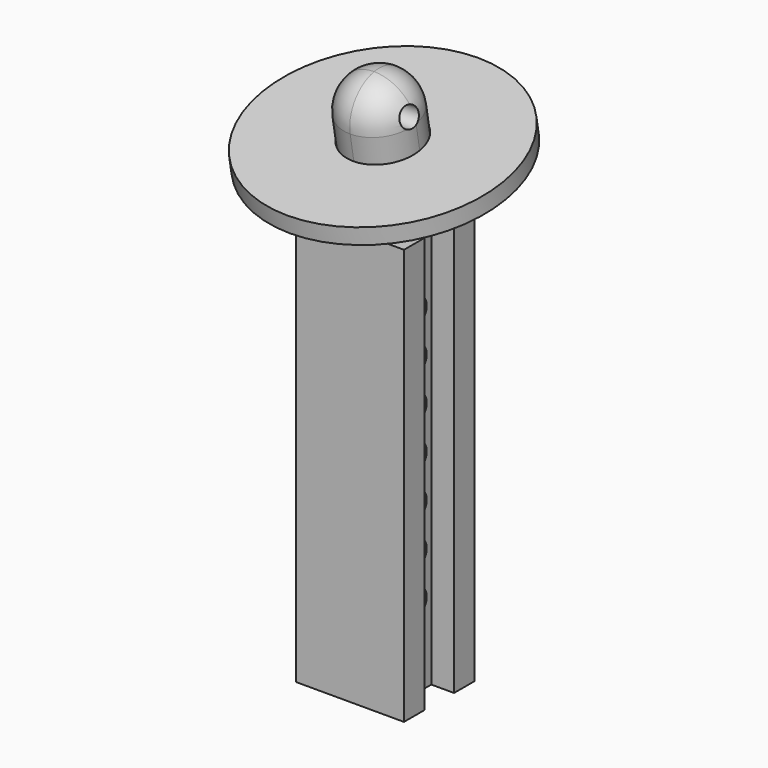
from build123d import *

# Parameters (mm, degrees)
F1_DEPTH     = 37.084
F3_DEPTH     = 25.4
F4_W         = 0.508
F4_H         = 3.302
F5_DEPTH     = 5.08
F6_T1_DEPTH  = 46.2057312575
F7_T1_DEPTH  = 13.1558517876
F7_T3_DEPTH  = 11.991388407
F9_DEPTH     = 7.112
F8_R         = 10.795
F10_DEPTH    = 1.524
F11_R        = 0.889
F12_DEPTH    = 25.4
F13_T1_DEPTH = 15.33525
F14_DEPTH    = 1.524
F15_T2_ANGLE = 89.9999999992
F15_T4_ANGLE = 90.0000000051
F15_T6_ANGLE = 89.9999999932
F15_T8_ANGLE = 89.9999999992


# Not quite as in the source:
# - a fillet or chamfer that OpenCascade refuses, or shapes differently, is made with other operations: its cross-section is extruded or revolved along the edge and cut away or added
# - a feature names something its author has since deleted; it is built from what else it names


with BuildPart() as f1:
    # F0 (on Top) → F1 (new body)
    with BuildSketch(Plane.XY):
        Polygon((13.1025131665, -0.5368698436), (3.4505131665, -0.5368698436), (3.4505131665, -2.8228698436), (5.4825131665, -2.8228698436), (5.4825131665, -6.1248698436), (3.4505131665, -6.1248698436), (3.4505131665, -8.4108698436), (13.1025131665, -8.4108698436), (13.1025131665, -6.1248698436), (11.0705131665, -6.1248698436), (11.0705131665, -2.8228698436), (13.1025131665, -2.8228698436), align=None)
    extrude(amount=F1_DEPTH)

    # F2 (on face) → F3 (cut)
    with BuildSketch(Plane.YZ.offset(11.0705131665)):
        with BuildLine():
            Line((-4.4738698436, 29.972), (-4.4738698436, 31.115))
            ThreePointArc((-4.4738698436, 31.115), (-5.6168698436, 29.972), (-4.4738698436, 28.829))
            Line((-4.4738698436, 28.829), (-4.4738698436, 29.972))
        make_face()
        with BuildLine():
            ThreePointArc((-4.4738698436, 28.829), (-3.6656467927, 29.1637769491), (-3.3308698436, 29.972))
            ThreePointArc((-3.3308698436, 29.972), (-3.6656467927, 30.7802230509), (-4.4738698436, 31.115))
            Line((-4.4738698436, 31.115), (-4.4738698436, 29.972))
            Line((-4.4738698436, 29.972), (-4.4738698436, 28.829))
        make_face()
        with BuildLine():
            ThreePointArc((-3.3308698436, 26.162), (-3.6656467927, 26.9702230509), (-4.4738698436, 27.305))
            Line((-4.4738698436, 27.305), (-4.4738698436, 26.162))
            Line((-4.4738698436, 26.162), (-4.4738698436, 25.019))
            ThreePointArc((-4.4738698436, 25.019), (-3.6656467927, 25.3537769491), (-3.3308698436, 26.162))
        make_face()
        with BuildLine():
            Line((-4.4738698436, 26.162), (-4.4738698436, 27.305))
            ThreePointArc((-4.4738698436, 27.305), (-5.6168698436, 26.162), (-4.4738698436, 25.019))
            Line((-4.4738698436, 25.019), (-4.4738698436, 26.162))
        make_face()
        with BuildLine():
            Line((-4.4738698436, 22.352), (-4.4738698436, 23.495))
            ThreePointArc((-4.4738698436, 23.495), (-5.6168698436, 22.352), (-4.4738698436, 21.209))
            Line((-4.4738698436, 21.209), (-4.4738698436, 22.352))
        make_face()
        with BuildLine():
            ThreePointArc((-3.3308698436, 22.352), (-3.6656467927, 23.1602230509), (-4.4738698436, 23.495))
            Line((-4.4738698436, 23.495), (-4.4738698436, 22.352))
            Line((-4.4738698436, 22.352), (-4.4738698436, 21.209))
            ThreePointArc((-4.4738698436, 21.209), (-3.6656467927, 21.5437769491), (-3.3308698436, 22.352))
        make_face()
        with BuildLine():
            ThreePointArc((-3.3308698436, 18.542), (-3.6656467927, 19.3502230509), (-4.4738698436, 19.685))
            Line((-4.4738698436, 19.685), (-4.4738698436, 18.542))
            Line((-4.4738698436, 18.542), (-4.4738698436, 17.399))
            ThreePointArc((-4.4738698436, 17.399), (-3.6656467927, 17.7337769491), (-3.3308698436, 18.542))
        make_face()
        with BuildLine():
            Line((-4.4738698436, 18.542), (-4.4738698436, 19.685))
            ThreePointArc((-4.4738698436, 19.685), (-5.6168698436, 18.542), (-4.4738698436, 17.399))
            Line((-4.4738698436, 17.399), (-4.4738698436, 18.542))
        make_face()
        with BuildLine():
            Line((-4.4738698436, 14.732), (-4.4738698436, 15.875))
            ThreePointArc((-4.4738698436, 15.875), (-5.6168698436, 14.732), (-4.4738698436, 13.589))
            Line((-4.4738698436, 13.589), (-4.4738698436, 14.732))
        make_face()
        with BuildLine():
            ThreePointArc((-3.3308698436, 14.732), (-3.6656467927, 15.5402230509), (-4.4738698436, 15.875))
            Line((-4.4738698436, 15.875), (-4.4738698436, 14.732))
            Line((-4.4738698436, 14.732), (-4.4738698436, 13.589))
            ThreePointArc((-4.4738698436, 13.589), (-3.6656467927, 13.9237769491), (-3.3308698436, 14.732))
        make_face()
        with BuildLine():
            Line((-4.4738698436, 10.922), (-4.4738698436, 9.779))
            ThreePointArc((-4.4738698436, 9.779), (-3.6656467927, 10.1137769491), (-3.3308698436, 10.922))
            ThreePointArc((-3.3308698436, 10.922), (-3.6656467927, 11.7302230509), (-4.4738698436, 12.065))
            Line((-4.4738698436, 12.065), (-4.4738698436, 10.922))
        make_face()
        with BuildLine():
            ThreePointArc((-4.4738698436, 12.065), (-5.6168698436, 10.922), (-4.4738698436, 9.779))
            Line((-4.4738698436, 9.779), (-4.4738698436, 10.922))
            Line((-4.4738698436, 10.922), (-4.4738698436, 12.065))
        make_face()
        with BuildLine():
            ThreePointArc((-4.4738698436, 8.255), (-5.6168698436, 7.112), (-4.4738698436, 5.969))
            Line((-4.4738698436, 5.969), (-4.4738698436, 7.112))
            Line((-4.4738698436, 7.112), (-4.4738698436, 8.255))
        make_face()
        with BuildLine():
            Line((-4.4738698436, 7.112), (-4.4738698436, 5.969))
            ThreePointArc((-4.4738698436, 5.969), (-3.6656467927, 6.3037769491), (-3.3308698436, 7.112))
            ThreePointArc((-3.3308698436, 7.112), (-3.6656467927, 7.9202230509), (-4.4738698436, 8.255))
            Line((-4.4738698436, 8.255), (-4.4738698436, 7.112))
        make_face()
    extrude(amount=-F3_DEPTH, mode=Mode.SUBTRACT)

    # F4 (on face) → F5 (join)
    with BuildSketch(Plane.XY.offset(37.084)):
        Polygon((11.5785131665, -2.8228698436), (11.5785131665, -1.1718698436), (4.9745131665, -1.1718698436), (4.9745131665, -2.8228698436), (5.4825131665, -2.8228698436), (5.4825131665, -6.1248698436), (4.9745131665, -6.1248698436), (4.9745131665, -7.7758698436), (11.5785131665, -7.7758698436), (11.5785131665, -6.1248698436), (11.0705131665, -6.1248698436), (11.0705131665, -2.8228698436), align=None)
        with Locations((5.2285131665, -4.4738698436)):
            Rectangle(F4_W, F4_H)
        with Locations((11.3245131665, -4.4738698436)):
            Rectangle(F4_W, F4_H)
    extrude(amount=F5_DEPTH)

    # F6: chamfer of 7.62 x 1.343611593 on 1 edges, made by hand

    # F6_s2 → F6_t1 (cut)
    with BuildSketch(Plane.YZ.offset(-14.8263524622)):
        Polygon((-7.7758698436, 40.820388407), (-0.1558698436, 42.164), (-7.7758698436, 42.164), align=None)
    extrude(amount=F6_T1_DEPTH, mode=Mode.SUBTRACT)

    # F7: fillet of radius 3.302 on 4 edges, made by hand

    # F7_s2 → F7_t1 (cut)
    with BuildSketch(Plane.XY.offset(37.084)):
        with BuildLine():
            ThreePointArc((8.2765131665, -1.1718698436), (5.941646575, -2.1390032521), (4.9745131665, -4.4738698436))
            Line((4.9745131665, -4.4738698436), (4.9745131665, -1.1718698436))
            Line((4.9745131665, -1.1718698436), (8.2765131665, -1.1718698436))
        make_face()
        with BuildLine():
            ThreePointArc((11.5785131665, -4.4738698436), (10.611379758, -2.1390032521), (8.2765131665, -1.1718698436))
            Line((8.2765131665, -1.1718698436), (11.5785131665, -1.1718698436))
            Line((11.5785131665, -1.1718698436), (11.5785131665, -4.4738698436))
        make_face()
    extrude(amount=F7_T1_DEPTH, mode=Mode.SUBTRACT)

    # F7_s4 → F7_t3 (cut)
    with BuildSketch(Plane.XY.offset(37.084)):
        with BuildLine():
            ThreePointArc((11.5785131665, -4.4738698436), (10.611379758, -6.8087364351), (8.2765131665, -7.7758698436))
            Line((8.2765131665, -7.7758698436), (11.5785131665, -7.7758698436))
            Line((11.5785131665, -7.7758698436), (11.5785131665, -4.4738698436))
        make_face()
        with BuildLine():
            ThreePointArc((4.9745131665, -4.4738698436), (5.941646575, -6.8087364351), (8.2765131665, -7.7758698436))
            Line((8.2765131665, -7.7758698436), (4.9745131665, -7.7758698436))
            Line((4.9745131665, -7.7758698436), (4.9745131665, -4.4738698436))
        make_face()
    extrude(amount=F7_T3_DEPTH, mode=Mode.SUBTRACT)

    # F8 (on face) → F9 (join)
    with BuildSketch(Plane(origin=(0, -7.2151687125, 40.9192551445), x_dir=(1, 0, 0), z_dir=(0, -0.1736481777, 0.984807753))):
        with BuildLine():
            add(Edge.make_bspline(
                [(7.6362341738, 6.0728878226), (5.2044151134, 5.584804343), (4.9872131665, 3.0773770998)],
                knots=[3.3505596509, 3.3505596509, 3.3505596509, 4.6166197938, 4.6166197938, 4.6166197938], degree=2, weights=[0.9324383972, 0.7591771847, 0.9664629106]))
            Line((7.6362341738, 6.0728878226), (4.9872131665, 6.0728878226))
            Line((4.9872131665, 6.0728878226), (4.9872131665, 3.0773770998))
        make_face()
        with BuildLine():
            Line((11.5658131665, 3.0773771001), (11.5658131665, 6.0728878226))
            Line((11.5658131665, 6.0728878226), (8.9167921592, 6.0728878226))
            add(Edge.make_bspline(
                [(11.5658131665, 3.0773771001), (11.3486112194, 5.5848043431), (8.9167921592, 6.0728878226)],
                knots=[1.6665655135, 1.6665655135, 1.6665655135, 2.9326256563, 2.9326256563, 2.9326256563], degree=2, weights=[0.9664629106, 0.7591771847, 0.9324383972]))
        make_face()
        with BuildLine():
            Line((11.5658131665, -0.5057121774), (11.5658131665, 2.4897985451))
            add(Edge.make_bspline(
                [(8.9167921595, -0.5057121774), (11.3486112194, -0.0176286977), (11.5658131665, 2.4897985451)],
                knots=[0.2089669974, 0.2089669974, 0.2089669974, 1.4750271401, 1.4750271401, 1.4750271401], degree=2, weights=[0.9324383972, 0.7591771848, 0.9664629106]))
            Line((8.9167921595, -0.5057121774), (11.5658131665, -0.5057121774))
        make_face()
        with BuildLine():
            add(Edge.make_bspline(
                [(4.9872131665, 2.4897985454), (5.2044151134, -0.0176286976), (7.6362341735, -0.5057121774)],
                knots=[4.808158167, 4.808158167, 4.808158167, 6.0742183098, 6.0742183098, 6.0742183098], degree=2, weights=[0.9664629106, 0.7591771847, 0.9324383972]))
            Line((4.9872131665, 2.4897985454), (4.9872131665, -0.5057121774))
            Line((4.9872131665, -0.5057121774), (7.6362341735, -0.5057121774))
        make_face()
        with BuildLine():
            add(Edge.make_bspline(
                [(11.5658131665, 3.0773771001), (11.3486112194, 5.5848043431), (8.9167921592, 6.0728878226)],
                knots=[1.6665655135, 1.6665655135, 1.6665655135, 2.9326256563, 2.9326256563, 2.9326256563], degree=2, weights=[0.9664629106, 0.7591771847, 0.9324383972]))
            Line((8.9167921592, 6.0728878226), (7.6362341738, 6.0728878226))
            add(Edge.make_bspline(
                [(7.6362341738, 6.0728878226), (5.2044151134, 5.584804343), (4.9872131665, 3.0773770998)],
                knots=[3.3505596509, 3.3505596509, 3.3505596509, 4.6166197938, 4.6166197938, 4.6166197938], degree=2, weights=[0.9324383972, 0.7591771847, 0.9664629106]))
            Line((4.9872131665, 3.0773770998), (4.9872131665, 2.4897985454))
            add(Edge.make_bspline(
                [(4.9872131665, 2.4897985454), (5.2044151134, -0.0176286976), (7.6362341735, -0.5057121774)],
                knots=[4.808158167, 4.808158167, 4.808158167, 6.0742183098, 6.0742183098, 6.0742183098], degree=2, weights=[0.9664629106, 0.7591771847, 0.9324383972]))
            Line((7.6362341735, -0.5057121774), (8.9167921595, -0.5057121774))
            add(Edge.make_bspline(
                [(8.9167921595, -0.5057121774), (11.3486112194, -0.0176286977), (11.5658131665, 2.4897985451)],
                knots=[0.2089669974, 0.2089669974, 0.2089669974, 1.4750271401, 1.4750271401, 1.4750271401], degree=2, weights=[0.9324383972, 0.7591771848, 0.9664629106]))
            Line((11.5658131665, 2.4897985451), (11.5658131665, 3.0773771001))
        make_face()
    extrude(amount=F9_DEPTH)

    # F11 (on face) → F12 (cut)
    with BuildSketch(Plane.YZ.offset(11.5658131665)):
        with Locations((-5.6265112944, 45.809186995)):
            Circle(F11_R)
    extrude(amount=-F12_DEPTH, mode=Mode.SUBTRACT)

    # F13: fillet of radius 3.2893 on 4 edges, made by hand

    # F13_s2 → F13_t1 (cut)
    with BuildSketch(Plane(origin=(0, -7.2151687125, 40.9192551445), x_dir=(1, 0, 0), z_dir=(0, -0.1736481777, 0.984807753))):
        with BuildLine():
            ThreePointArc((11.5658131665, 2.7835878226), (10.6023995018, 0.4577014873), (8.2765131665, -0.5057121774))
            Line((8.2765131665, -0.5057121774), (11.5658131665, -0.5057121774))
            Line((11.5658131665, -0.5057121774), (11.5658131665, 2.7835878226))
        make_face()
        with BuildLine():
            ThreePointArc((4.9872131665, 2.7835878226), (5.9506268311, 0.4577014873), (8.2765131665, -0.5057121774))
            Line((8.2765131665, -0.5057121774), (4.9872131665, -0.5057121774))
            Line((4.9872131665, -0.5057121774), (4.9872131665, 2.7835878226))
        make_face()
        with BuildLine():
            ThreePointArc((8.2765131665, 6.0728878226), (10.6023995018, 5.109474158), (11.5658131665, 2.7835878226))
            Line((11.5658131665, 2.7835878226), (11.5658131665, 6.0728878226))
            Line((11.5658131665, 6.0728878226), (8.2765131665, 6.0728878226))
        make_face()
        with BuildLine():
            ThreePointArc((8.2765131665, 6.0728878226), (5.9506268311, 5.109474158), (4.9872131665, 2.7835878226))
            Line((4.9872131665, 2.7835878226), (4.9872131665, 6.0728878226))
            Line((4.9872131665, 6.0728878226), (8.2765131665, 6.0728878226))
        make_face()
    extrude(amount=F13_T1_DEPTH, mode=Mode.SUBTRACT)

    # F15: fillet of radius 3.2893 on 4 edges, made by hand

    # F15_s1 → F15_t2 (revolve, cut)
    with BuildSketch(Plane.YZ.offset(8.2765131665)):
        with BuildLine():
            ThreePointArc((-1.8983465904, 45.7384256455), (-3.2510097603, 47.861681514), (-5.7088556832, 48.4065728367))
            Line((-5.7088556832, 48.4065728367), (-2.4695275412, 48.9777537875))
            Line((-2.4695275412, 48.9777537875), (-1.8983465904, 45.7384256455))
        make_face()
    revolve(axis=Axis((8.2765131665, -5.7088556832, 48.4065728367), (0, 0.1736481777, -0.984807753)), revolution_arc=F15_T2_ANGLE, mode=Mode.SUBTRACT)

    # F15_s3 → F15_t4 (revolve, cut)
    with BuildSketch(Plane(origin=(-1e-10, 2.7412988687, 0.4833649527), x_dir=(1, 0, 0), z_dir=(0, -0.984807753, -0.1736481777))):
        with BuildLine():
            ThreePointArc((4.9872131663, 45.3732006123), (5.9506268309, 47.6990869477), (8.2765131662, 48.6625006124))
            Line((8.2765131662, 48.6625006124), (4.9872131662, 48.6625006123))
            Line((4.9872131662, 48.6625006123), (4.9872131663, 45.3732006123))
        make_face()
    revolve(axis=Axis((8.2765131664, -5.708855683, 48.4065728367), (0, 0.1736481777, -0.984807753)), revolution_arc=F15_T4_ANGLE, mode=Mode.SUBTRACT)

    # F15_s5 → F15_t6 (revolve, cut)
    with BuildSketch(Plane(origin=(2e-10, 2.7412988696, 0.4833649529), x_dir=(-1, 1e-10, 0), z_dir=(1e-10, 0.984807753, 0.1736481777))):
        with BuildLine():
            ThreePointArc((-11.5658131668, 45.3732006122), (-10.6023995022, 47.6990869475), (-8.2765131668, 48.6625006122))
            Line((-8.2765131668, 48.6625006122), (-11.5658131668, 48.6625006122))
            Line((-11.5658131668, 48.6625006122), (-11.5658131668, 45.3732006122))
        make_face()
    revolve(axis=Axis((8.2765131663, -5.708855683, 48.4065728368), (0, 0.1736481777, -0.984807753)), revolution_arc=F15_T6_ANGLE, mode=Mode.SUBTRACT)

    # F15_s7 → F15_t8 (revolve, cut)
    with BuildSketch(Plane.YZ.offset(8.2765131665)):
        with BuildLine():
            ThreePointArc((-8.3770028743, 44.5960637439), (-7.8321115516, 47.0539096668), (-5.7088556832, 48.4065728367))
            Line((-5.7088556832, 48.4065728367), (-8.9481838251, 47.8353918859))
            Line((-8.9481838251, 47.8353918859), (-8.3770028743, 44.5960637439))
        make_face()
    revolve(axis=Axis((8.2765131665, -5.7088556831, 48.4065728367), (0, 0.1736481777, -0.984807753)), revolution_arc=F15_T8_ANGLE, mode=Mode.SUBTRACT)


with BuildPart() as f10:
    # F8 (on face) → F10 (new body)
    with BuildSketch(Plane(origin=(0, -7.2151687125, 40.9192551445), x_dir=(1, 0, 0), z_dir=(0, -0.1736481777, 0.984807753))):
        with Locations((8.2765131665, 2.7835878226)):
            Circle(F8_R)
        with BuildLine():
            Line((8.9167921592, 6.0728878226), (11.5658131665, 6.0728878226))
            Line((11.5658131665, 6.0728878226), (11.5658131665, 3.0773771001))
            add(Edge.make_bspline(
                [(11.5785131665, 2.7835878226), (11.5785131665, 2.9307654953), (11.5658131665, 3.0773771001)],
                knots=[1.5707963268, 1.5707963268, 1.5707963268, 1.6665655135, 1.6665655135, 1.6665655135], degree=2, weights=[1, 0.9821427228, 0.9664629106]))
            add(Edge.make_bspline(
                [(11.5658131665, 2.4897985451), (11.5785131665, 2.6364101498), (11.5785131665, 2.7835878226)],
                knots=[1.4750271401, 1.4750271401, 1.4750271401, 1.5707963268, 1.5707963268, 1.5707963268], degree=2, weights=[0.9664629106, 0.9821427228, 1]))
            Line((11.5658131665, 2.4897985451), (11.5658131665, -0.5057121774))
            Line((11.5658131665, -0.5057121774), (8.9167921595, -0.5057121774))
            add(Edge.make_bspline(
                [(8.2765131665, -0.5693508499), (8.5997198898, -0.5693508499), (8.9167921595, -0.5057121774)],
                knots=[0, 0, 0, 0.2089669974, 0.2089669974, 0.2089669974], degree=2, weights=[1, 0.9610356763, 0.9324383972]))
            add(Edge.make_bspline(
                [(7.6362341735, -0.5057121774), (7.9533064432, -0.5693508499), (8.2765131665, -0.5693508499)],
                knots=[6.0742183098, 6.0742183098, 6.0742183098, 6.2831853072, 6.2831853072, 6.2831853072], degree=2, weights=[0.9324383972, 0.9610356763, 1]))
            Line((7.6362341735, -0.5057121774), (4.9872131665, -0.5057121774))
            Line((4.9872131665, -0.5057121774), (4.9872131665, 2.4897985454))
            add(Edge.make_bspline(
                [(4.9745131665, 2.7835878226), (4.9745131665, 2.63641015), (4.9872131665, 2.4897985454)],
                knots=[4.7123889804, 4.7123889804, 4.7123889804, 4.808158167, 4.808158167, 4.808158167], degree=2, weights=[1, 0.9821427229, 0.9664629106]))
            add(Edge.make_bspline(
                [(4.9872131665, 3.0773770998), (4.9745131665, 2.9307654952), (4.9745131665, 2.7835878226)],
                knots=[4.6166197938, 4.6166197938, 4.6166197938, 4.7123889804, 4.7123889804, 4.7123889804], degree=2, weights=[0.9664629106, 0.9821427229, 1]))
            Line((4.9872131665, 3.0773770998), (4.9872131665, 6.0728878226))
            Line((4.9872131665, 6.0728878226), (7.6362341738, 6.0728878226))
            add(Edge.make_bspline(
                [(8.2765131665, 6.136526495), (7.9533064433, 6.136526495), (7.6362341738, 6.0728878226)],
                knots=[3.1415926536, 3.1415926536, 3.1415926536, 3.3505596509, 3.3505596509, 3.3505596509], degree=2, weights=[1, 0.9610356763, 0.9324383972]))
            add(Edge.make_bspline(
                [(8.9167921592, 6.0728878226), (8.5997198897, 6.136526495), (8.2765131665, 6.136526495)],
                knots=[2.9326256563, 2.9326256563, 2.9326256563, 3.1415926536, 3.1415926536, 3.1415926536], degree=2, weights=[0.9324383972, 0.9610356763, 1]))
        make_face(mode=Mode.SUBTRACT)
    extrude(amount=F10_DEPTH)

    # F8 (on face) → F14 (join)
    with BuildSketch(Plane(origin=(0, -7.2151687125, 40.9192551445), x_dir=(1, 0, 0), z_dir=(0, -0.1736481777, 0.984807753))):
        with BuildLine():
            Line((11.5658131665, 3.0773771001), (11.5658131665, 6.0728878226))
            Line((11.5658131665, 6.0728878226), (8.9167921592, 6.0728878226))
            add(Edge.make_bspline(
                [(11.5658131665, 3.0773771001), (11.3486112194, 5.5848043431), (8.9167921592, 6.0728878226)],
                knots=[1.6665655135, 1.6665655135, 1.6665655135, 2.9326256563, 2.9326256563, 2.9326256563], degree=2, weights=[0.9664629106, 0.7591771847, 0.9324383972]))
        make_face()
        with BuildLine():
            add(Edge.make_bspline(
                [(7.6362341738, 6.0728878226), (5.2044151134, 5.584804343), (4.9872131665, 3.0773770998)],
                knots=[3.3505596509, 3.3505596509, 3.3505596509, 4.6166197938, 4.6166197938, 4.6166197938], degree=2, weights=[0.9324383972, 0.7591771847, 0.9664629106]))
            Line((7.6362341738, 6.0728878226), (4.9872131665, 6.0728878226))
            Line((4.9872131665, 6.0728878226), (4.9872131665, 3.0773770998))
        make_face()
        with BuildLine():
            add(Edge.make_bspline(
                [(4.9872131665, 2.4897985454), (5.2044151134, -0.0176286976), (7.6362341735, -0.5057121774)],
                knots=[4.808158167, 4.808158167, 4.808158167, 6.0742183098, 6.0742183098, 6.0742183098], degree=2, weights=[0.9664629106, 0.7591771847, 0.9324383972]))
            Line((4.9872131665, 2.4897985454), (4.9872131665, -0.5057121774))
            Line((4.9872131665, -0.5057121774), (7.6362341735, -0.5057121774))
        make_face()
        with BuildLine():
            Line((11.5658131665, -0.5057121774), (11.5658131665, 2.4897985451))
            add(Edge.make_bspline(
                [(8.9167921595, -0.5057121774), (11.3486112194, -0.0176286977), (11.5658131665, 2.4897985451)],
                knots=[0.2089669974, 0.2089669974, 0.2089669974, 1.4750271401, 1.4750271401, 1.4750271401], degree=2, weights=[0.9324383972, 0.7591771848, 0.9664629106]))
            Line((8.9167921595, -0.5057121774), (11.5658131665, -0.5057121774))
        make_face()
    extrude(amount=F14_DEPTH)


solid = Compound([f1.part, f10.part])
